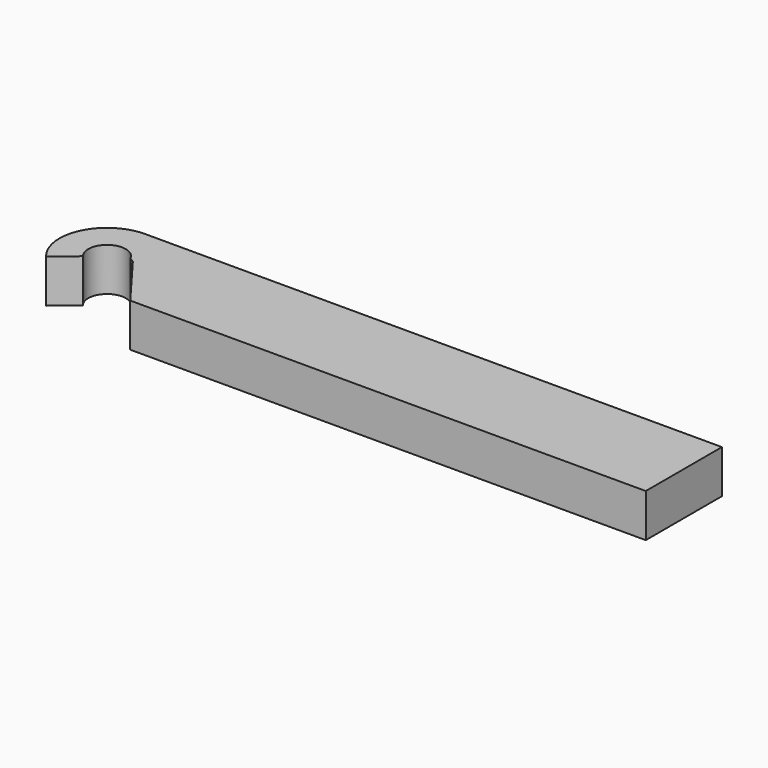
from build123d import *

# Parameters (mm, degrees)
F1_DEPTH    = 3
F2_T4_DEPTH = 7.0269593276


# Not quite as in the source:
# - a fillet or chamfer that OpenCascade refuses, or shapes differently, is made with other operations: its cross-section is extruded or revolved along the edge and cut away or added


with BuildPart() as f1:
    # F0 (on Top) → F1 (new body)
    with BuildSketch(Plane.XY):
        with BuildLine():
            ThreePointArc((-40.9958577761, -0.8356238926), (-40.4446261863, 1.221600407), (-38.7, 0))
            Line((-38.7, 0), (-38.2265411317, 0))
            Line((-38.2265411317, 0), (-36.7, 0))
            ThreePointArc((-36.7, 0), (-36.7956166893, -0.7886238635), (-37.076925817, -1.5315473615))
            Line((-37.076925817, -1.5315473615), (-35.7494838536, -3.3))
            Line((-35.7494838536, -3.3), (0, -3.3))
            Line((0, -3.3), (0, 0))
            Line((0, 0), (0, 3.3))
            Line((0, 3.3), (-40, 3.3))
            ThreePointArc((-40, 3.3), (-42.9908156972, 1.3946402637), (-42.5279466623, -2.121199112))
            Line((-42.5279466623, -2.121199112), (-40.9958577761, -0.8356238926))
        make_face()
        with BuildLine():
            Line((-36.7, 0), (-38.2265411317, 0))
            Line((-38.2265411317, 0), (-37.076925817, -1.5315473615))
            ThreePointArc((-37.076925817, -1.5315473615), (-36.7956166893, -0.7886238635), (-36.7, 0))
        make_face()
    extrude(amount=F1_DEPTH)

    # F2: chamfer of 1 on 1 edges, made by hand


with BuildPart() as f2_tool2:
    # F2_s3 → F2_t4 (new body)
    with BuildSketch(Plane.XY.offset(-2.0134796638)):
        with BuildLine():
            Line((-38.8293039248, 0.5652173913), (-37.9287684823, 0))
            Line((-37.9287684823, 0), (-38.7, 0))
            ThreePointArc((-38.7, 0), (-38.7360904804, 0.3041919232), (-38.8293039248, 0.5652173913))
        make_face()
    extrude(amount=F2_T4_DEPTH)

    split(bisect_by=Plane(origin=(-24.4503471764, -18.3530031596, 0), x_dir=(0, 0, 1), z_dir=(-0.7997606156, -0.6003190466, 0)), keep=Keep.TOP)


with BuildPart() as f1_1:
    add(f1.part)

    # F2_t1: cut F2_tool2
    add(f2_tool2.part, mode=Mode.SUBTRACT)


solid = f1_1.part
